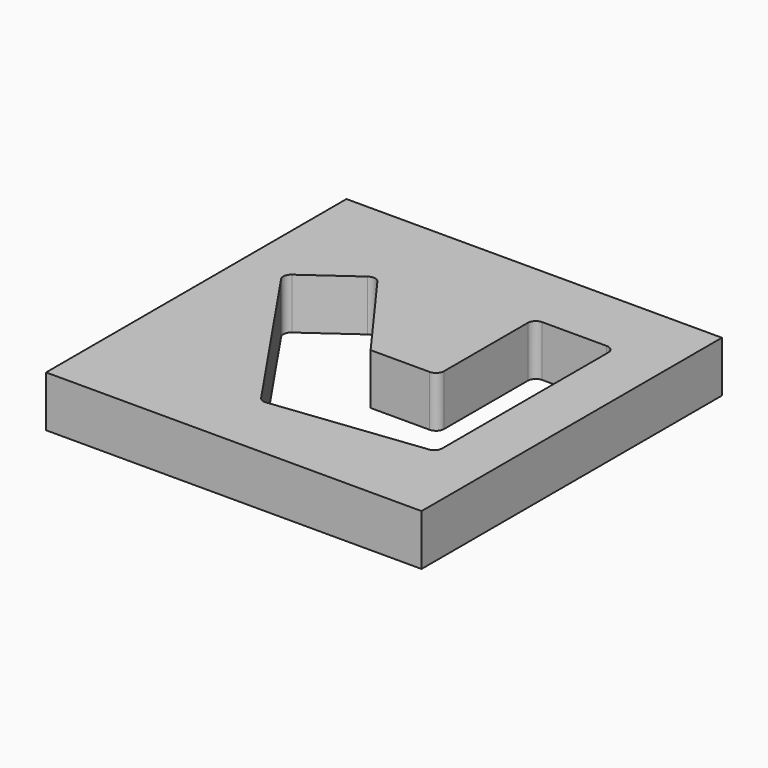
from build123d import *

# Parameters (mm, degrees)
F0_W     = 140
F0_H     = 140
F1_DEPTH = 19
F3_DEPTH = 20
F4_R     = 3


# Not quite as in the source:
# - a feature names something its author has since deleted; it is built from what else it names


with BuildPart() as f1:
    # F0 (on Top) → F1 (new body)
    with BuildSketch(Plane.XY):
        Rectangle(F0_W, F0_H)
    extrude(amount=F1_DEPTH)

    # F2 (on face) → F3 (cut)
    with BuildSketch(Plane.XY.offset(19)):
        Polygon((20, 0), (0, 0), (-5, 0), (-32.2085873907, 37.4088223177), (-55, 21.1437827766), (-10, -45), (50, -38), (50, 45), (20, 45), align=None)
    extrude(amount=-F3_DEPTH, mode=Mode.SUBTRACT)

    # F4
    f4_edges = [f1.edges().sort_by_distance(p)[0] for p in [
        (50, -38, 9.5),
        (50, 45, 9.5),
        (20, 45, 9.5),
        (20, 0, 9.5),
        (-55, 21.143783, 9.5),
        (-10, -45, 9.5),
        (-32.208587, 37.408822, 9.5),
    ]]
    fillet(f4_edges, radius=F4_R)


solid = f1.part
